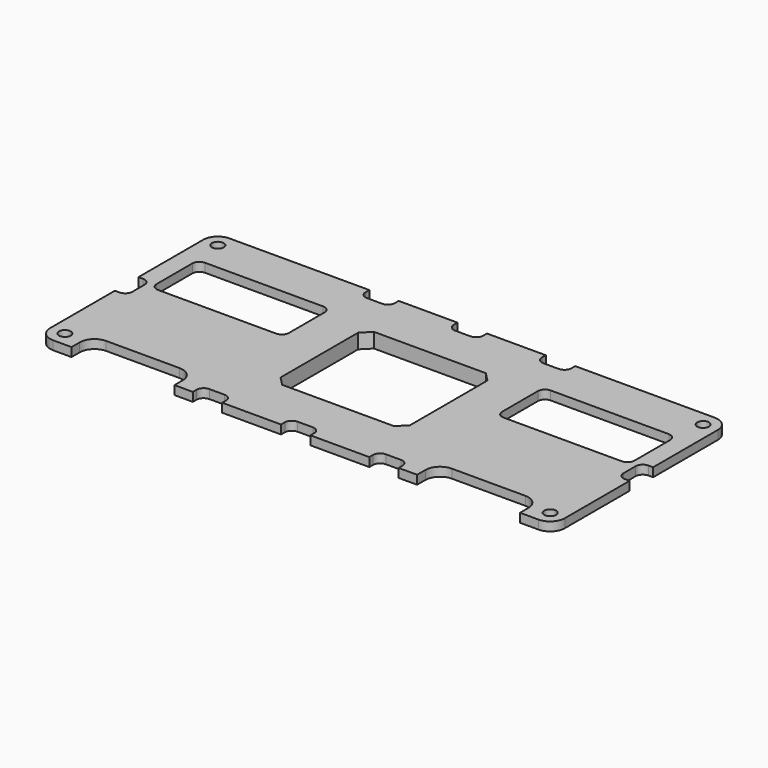
from build123d import *

# Parameters (mm, degrees)
F1_DEPTH      = 3
F2_W          = 4
F2_H          = 10
F2_W_2        = 70
F2_H_2        = 4
F3_DEPTH      = 20.4
F4_R          = 2
F5_DEPTH      = 25
F6_W          = 44
F6_H          = 39
F7_DEPTH      = 25
F9_DEPTH      = 25
F10_W         = 20
F10_H         = 4
F11_DEPTH     = 3
F12_W         = 45
F12_H         = 20
F13_DEPTH     = 25
F14_R         = 2.4142135624
F15_SIZE      = 3
F16_R         = 30
F17_DEPTH     = 2
F18_TEXT_SIZE = 16.6666666667
F19_DEPTH     = 0.5
F20_DEPTH     = 0.5


# Not quite as in the source:
# - Text() gives the source's letters only with a copy of the font that has no kerning and outlines rounded to 1/6400 em; it was checked with that copy


with BuildPart() as f1:
    # F0 (on Top) → F1 (new body)
    with BuildSketch(Plane.XY):
        with BuildLine():
            ThreePointArc((87.5, 32.5), (86.0355339059, 36.0355339059), (82.5, 37.5))
            Line((82.5, 37.5), (-82.5, 37.5))
            ThreePointArc((-82.5, 37.5), (-86.0355339059, 36.0355339059), (-87.5, 32.5))
            Line((-87.5, 32.5), (-87.5, -32.5))
            ThreePointArc((-87.5, -32.5), (-86.0355339059, -36.0355339059), (-82.5, -37.5))
            Line((-82.5, -37.5), (82.5, -37.5))
            ThreePointArc((82.5, -37.5), (86.0355339059, -36.0355339059), (87.5, -32.5))
            Line((87.5, -32.5), (87.5, 32.5))
        make_face()
    extrude(amount=F1_DEPTH)

    # F2 (on face) → F3 (cut)
    with BuildSketch(Plane.XY.offset(3)):
        with Locations((-85.5, 0)):
            Rectangle(F2_W, F2_H)
        with Locations((-89.5, 0)):
            Rectangle(F2_W, F2_H)
        with Locations((0, 35.5)):
            Rectangle(F2_W_2, F2_H_2)
        with Locations((0, 39.5)):
            Rectangle(F2_W_2, F2_H_2)
        with Locations((85.5, 0)):
            Rectangle(F2_W, F2_H)
        with Locations((89.5, 0)):
            Rectangle(F2_W, F2_H)
        with Locations((0, -35.5)):
            Rectangle(F2_W_2, F2_H_2)
        with Locations((0, -39.5)):
            Rectangle(F2_W_2, F2_H_2)
    extrude(amount=-F3_DEPTH, mode=Mode.SUBTRACT)

    # F4 (on face) → F5 (cut)
    with BuildSketch(Plane.XY.offset(3)):
        with Locations((-82.5, 32.5)):
            Circle(F4_R)
        with Locations((-82.5, -32.5)):
            Circle(F4_R)
        with Locations((82.5, 32.5)):
            Circle(F4_R)
        with Locations((82.5, -32.5)):
            Circle(F4_R)
    extrude(amount=-F5_DEPTH, mode=Mode.SUBTRACT)

    # F6 (on face) → F7 (cut)
    with BuildSketch(Plane.XY.offset(3)):
        Rectangle(F6_W, F6_H)
    extrude(amount=-F7_DEPTH, mode=Mode.SUBTRACT)

    # F8 (on face) → F9 (cut)
    with BuildSketch(Plane.XY.offset(3)):
        with BuildLine():
            Line((-76.25, -46), (-41.25, -46))
            Line((-41.25, -46), (-41.25, -34))
            ThreePointArc((-41.25, -34), (-42.7144660941, -30.4644660941), (-46.25, -29))
            Line((-46.25, -29), (-71.25, -29))
            ThreePointArc((-71.25, -29), (-74.7855339059, -30.4644660941), (-76.25, -34))
            Line((-76.25, -34), (-76.25, -46))
        make_face()
        with BuildLine():
            Line((41.25, -46), (76.25, -46))
            Line((76.25, -46), (76.25, -34))
            ThreePointArc((76.25, -34), (74.7855339059, -30.4644660941), (71.25, -29))
            Line((71.25, -29), (46.25, -29))
            ThreePointArc((46.25, -29), (42.7144660941, -30.4644660941), (41.25, -34))
            Line((41.25, -34), (41.25, -46))
        make_face()
    extrude(amount=-F9_DEPTH, mode=Mode.SUBTRACT)

    # F10 (on face) → F11 (join)
    with BuildSketch(Plane.XY.offset(3)):
        with Locations((-15, -35.5)):
            Rectangle(F10_W, F10_H)
        with Locations((15, -35.5)):
            Rectangle(F10_W, F10_H)
        with Locations((-15, -31.5)):
            Rectangle(F10_W, F10_H)
        with Locations((15, -31.5)):
            Rectangle(F10_W, F10_H)
        with Locations((-15, 31.5)):
            Rectangle(F10_W, F10_H)
        with Locations((-15, 35.5)):
            Rectangle(F10_W, F10_H)
        with Locations((15, 35.5)):
            Rectangle(F10_W, F10_H)
        with Locations((15, 31.5)):
            Rectangle(F10_W, F10_H)
    extrude(amount=-F11_DEPTH)

    # F12 (on face) → F13 (cut)
    with BuildSketch(Plane.XY.offset(3)):
        with Locations((-58.75, 12.5)):
            Rectangle(F12_W, F12_H)
        with Locations((58.75, 12.5)):
            Rectangle(F12_W, F12_H)
    extrude(amount=-F13_DEPTH, mode=Mode.SUBTRACT)

    # F14
    f14_edges = [f1.edges().sort_by_distance(p)[0] for p in [
        (-36.25, 22.5, 1.5),
        (-36.25, 2.5, 1.5),
        (-25, 33.5, 1.5),
        (-35, 33.5, 1.5),
        (-5, 33.5, 1.5),
        (5, 33.5, 1.5),
        (25, 33.5, 1.5),
        (35, 33.5, 1.5),
        (36.25, 22.5, 1.5),
        (36.25, 2.5, 1.5),
        (35, -33.5, 1.5),
        (25, -33.5, 1.5),
        (-5, -33.5, 1.5),
        (5, -33.5, 1.5),
        (-25, -33.5, 1.5),
        (-35, -33.5, 1.5),
        (83.5, 5, 1.5),
        (83.5, -5, 1.5),
        (-83.5, -5, 1.5),
        (-83.5, 5, 1.5),
        (-81.25, 2.5, 1.5),
        (-81.25, 22.5, 1.5),
        (81.25, 22.5, 1.5),
        (81.25, 2.5, 1.5),
    ]]
    fillet(f14_edges, radius=F14_R)

    # F15
    f15_edges = [f1.edges().sort_by_distance(p)[0] for p in [
        (-22, 19.5, 1.5),
        (22, 19.5, 1.5),
        (-22, -19.5, 1.5),
        (22, -19.5, 1.5),
    ]]
    chamfer(f15_edges, length=F15_SIZE)

    # F16 (on face) → F17 (join)
    with BuildSketch(Plane(origin=(0, 0, 0), x_dir=(1, 0, 0), z_dir=(0, 0, -1))):
        Circle(F16_R)
        Polygon((19, 19.5), (22, 16.5), (22, -16.5), (19, -19.5), (-19, -19.5), (-22, -16.5), (-22, 16.5), (-19, 19.5), align=None, mode=Mode.SUBTRACT)
    extrude(amount=F17_DEPTH)

    # F18 (on face) → F19 (cut)
    with BuildSketch(Plane(origin=(0, 0, 0), x_dir=(1, 0, 0), z_dir=(0, 0, -1))):
        with Locations((-82.71484375, 5.4912797455)):
            Text('VESC1', F18_TEXT_SIZE, font='Open Sans', font_style=FontStyle.BOLD, text_align=(TextAlign.LEFT, TextAlign.BOTTOM))
    extrude(amount=-F19_DEPTH, mode=Mode.SUBTRACT)

    # F18 (on face) → F20 (cut)
    with BuildSketch(Plane(origin=(0, 0, 0), x_dir=(1, 0, 0), z_dir=(0, 0, -1))):
        with Locations((33.7356770833, 4.8793592602)):
            Text('VESC2', F18_TEXT_SIZE, font='Open Sans', font_style=FontStyle.BOLD, text_align=(TextAlign.LEFT, TextAlign.BOTTOM))
    extrude(amount=-F20_DEPTH, mode=Mode.SUBTRACT)


solid = f1.part
